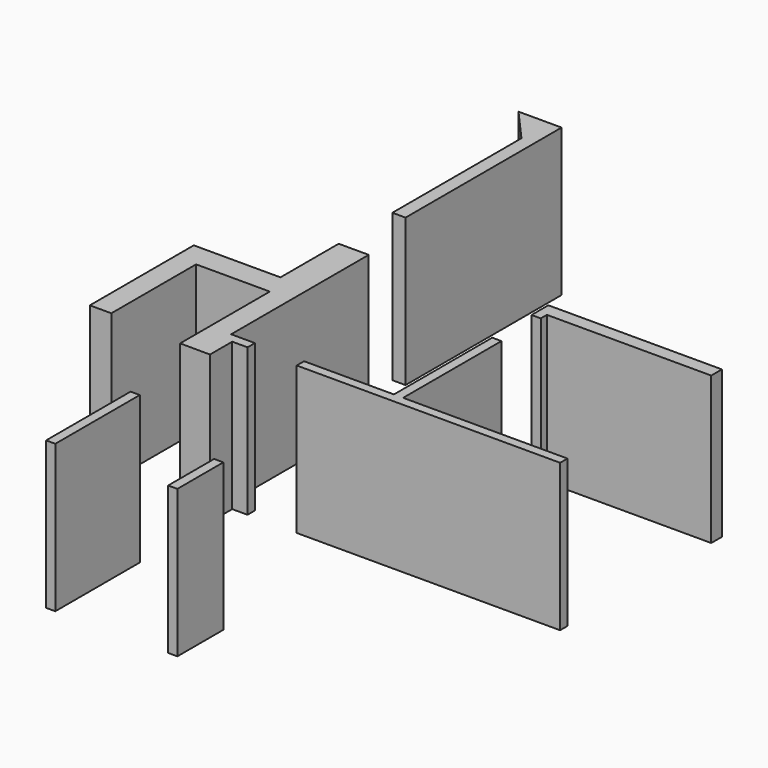
from build123d import *

# Parameters (mm, degrees)
F1_DEPTH = 2438.4
F0_W     = 152.4
F0_H     = 950.3680467606
F0_H_2   = 1746.8922138214


# Not quite as in the source:
# - the program builds the solid bodies; features that only make, move or delete a surface that nothing else refers to are left out


with BuildPart() as f1:
    # F0 (on Top) → F1 (new body)
    with BuildSketch(Plane.XY):
        Polygon((-3847.3440776825, 1188.7577511787), (-3847.3440776825, 1648.9702011108), (-3594.1724777222, 1648.9702011108), (-3594.1724777222, 1801.3702011108), (-3987.6942779541, 1801.3702011108), (-3987.6942779541, 4646.1702011108), (-4484.7030639648, 4646.1702011108), (-4484.7030639648, 3442.4197673798), (-5918.0942779541, 3442.4197673798), (-5918.0942779541, 3045.9702011108), (-5918.0942779541, 1293.3702011108), (-5562.4942779541, 1293.3702011108), (-5562.4942779541, 3045.9702011108), (-4343.2942779541, 3045.9702011108), (-4343.2942779541, 1191.7702011108), align=None)
    extrude(amount=F1_DEPTH)


with BuildPart() as f1b:
    # F0 (on Top) → F1, piece 2 (new body)
    with BuildSketch(Plane.XY):
        Polygon((-4267.0942779541, 5756.060754776), (-4267.0942779541, 8981.860754776), (-4979.4447412196, 8981.860754776), (-4484.7030639648, 8424.8667533997), (-4484.7030639648, 5930.2643890381), (-4484.7030639648, 5756.060754776), align=None)
    extrude(amount=F1_DEPTH)


with BuildPart() as f1c:
    # F0 (on Top) → F1, piece 3 (new body)
    with BuildSketch(Plane.XY):
        Polygon((-1142.8942779541, 4773.1702011108), (1574.9057220459, 4773.1702011108), (1574.9057220459, 4994.060754776), (-1295.2942779541, 4994.060754776), (-1295.2942779541, 4646.1702011108), (-1142.8942779541, 4646.1702011108), align=None)
    extrude(amount=F1_DEPTH)


with BuildPart() as f1d:
    # F0 (on Top) → F1, piece 4 (new body)
    with BuildSketch(Plane.XY):
        Polygon((-2781.3724777222, 1648.9702011108), (1574.9057220459, 1648.9702011108), (1574.9057220459, 1801.3702011108), (-1142.8942779541, 1801.3702011108), (-1142.8942779541, 3833.3702011108), (-1295.2942779541, 3833.3702011108), (-1295.2942779541, 1801.3702011108), (-2781.3724777222, 1801.3702011108), align=None)
    extrude(amount=F1_DEPTH)


with BuildPart() as f1e:
    # F0 (on Top) → F1, piece 5 (new body)
    with BuildSketch(Plane.XY):
        with Locations((-1904.8942779541, -1533.4457755089)):
            Rectangle(F0_W, F0_H)
    extrude(amount=F1_DEPTH)


with BuildPart() as f1f:
    # F0 (on Top) → F1, piece 6 (new body)
    with BuildSketch(Plane.XY):
        with Locations((-3923.5440776825, -1135.1836919785)):
            Rectangle(F0_W, F0_H_2)
    extrude(amount=F1_DEPTH)


solid = Compound([f1.part, f1b.part, f1c.part, f1d.part, f1e.part, f1f.part])
